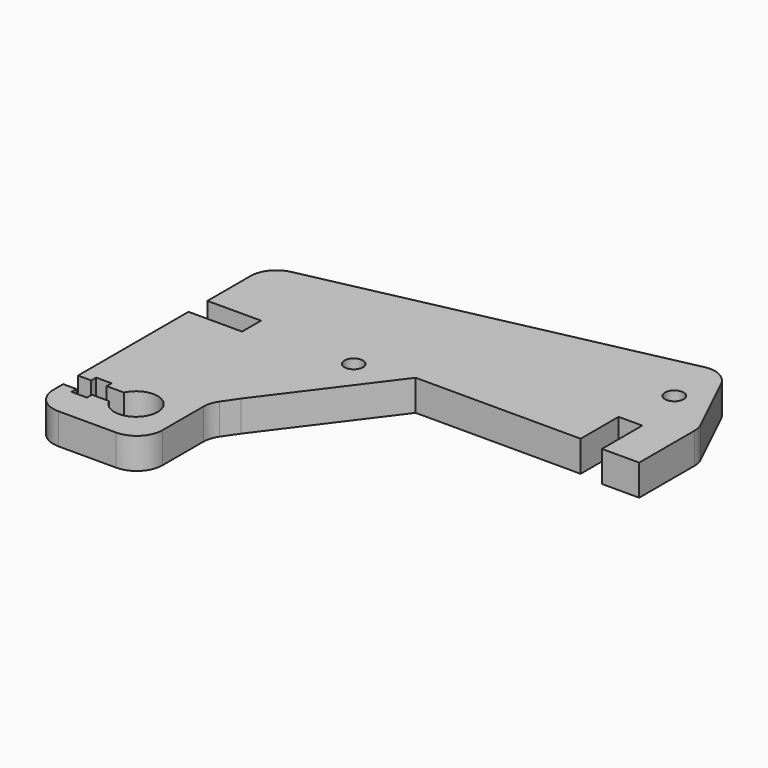
from build123d import *

# Parameters (mm, degrees)
F0_R     = 1.8
F1_DEPTH = 6


# Not quite as in the source:
# - a feature names something its author has since deleted; it is built from what else it names


with BuildPart() as f1:
    # F0 (on Top) → F1 (new body)
    with BuildSketch(Plane.XY):
        with BuildLine():
            ThreePointArc((-26.9197331922, -29.0044), (-22.202470707, -26.7069691338), (-18.925, -30.8044))
            ThreePointArc((-18.925, -30.8044), (-22.202470707, -34.9018308662), (-26.9197331922, -32.6044))
            Line((-26.9197331922, -32.6044), (-30.2622788846, -32.6044))
            Line((-30.2622788846, -32.6044), (-30.2622788846, -33.8044))
            Line((-30.2622788846, -33.8044), (-33.2622788846, -33.8044))
            Line((-33.2622788846, -33.8044), (-33.2622788846, -32.6044))
            Line((-33.2622788846, -32.6044), (-35.8254, -32.6044))
            Line((-35.8254, -32.6044), (-35.8254, -35.0044))
            ThreePointArc((-35.8254, -35.0044), (-34.3609339059, -38.5399339059), (-30.8254, -40.0044))
            Line((-30.8254, -40.0044), (-19.625, -40.0044))
            ThreePointArc((-19.625, -40.0044), (-16.0894660941, -38.5399339059), (-14.625, -35.0044))
            Line((-14.625, -35.0044), (-14.625, -25.0977827265))
            ThreePointArc((-14.625, -25.0977827265), (-14.400006794, -23.6147756066), (-13.7452759529, -22.2652350973))
            Line((-13.7452759529, -22.2652350973), (-11.8023123147, -19.4389644026))
            Line((-11.8023123147, -19.4389644026), (4.5746, 2.4))
            Line((4.5746, 2.4), (36.6099, 2.4))
            Line((36.6099, 2.4), (36.6099, 11.6009423509))
            Line((36.6099, 11.6009423509), (37.1099, 11.6009423509))
            Line((37.1099, 11.6009423509), (38.9099, 11.6009423509))
            Line((38.9099, 11.6009423509), (40.7099, 11.6009423509))
            Line((40.7099, 11.6009423509), (41.2099, 11.6009423509))
            Line((41.2099, 11.6009423509), (41.2099, 1.8140082314))
            Line((41.2099, 1.8140082314), (48.4484305441, 1.8140082314))
            Line((48.4484305441, 1.8140082314), (48.4484305441, 15.1736566274))
            ThreePointArc((48.4484305441, 15.1736566274), (48.3232531582, 16.2854589848), (47.9539887514, 17.341592337))
            Line((47.9539887514, 17.341592337), (41.9726020282, 29.7725357096))
            ThreePointArc((41.9726020282, 29.7725357096), (40.1857248711, 31.8008808947), (37.6042192016, 32.6027179373))
            ThreePointArc((37.6042192016, 32.6027179373), (37.1447174672, 32.5688699786), (36.6902824172, 32.4928679158))
            Line((36.6902824172, 32.4928679158), (-31.8765121651, 17.7491195886))
            ThreePointArc((-31.8765121651, 17.7491195886), (-34.7148447435, 16.0028605187), (-35.8254, 12.8608516729))
            Line((-35.8254, 12.8608516729), (-35.8254, 2.4))
            Line((-35.8254, 2.4), (-25.4254, 2.4))
            Line((-25.4254, 2.4), (-25.4254, 1.9))
            Line((-25.4254, 1.9), (-25.4254, -1.7))
            Line((-25.4254, -1.7), (-25.4254, -2.2))
            Line((-25.4254, -2.2), (-35.8254, -2.2))
            Line((-35.8254, -2.2), (-35.8254, -29.0044))
            Line((-35.8254, -29.0044), (-33.2622788846, -29.0044))
            Line((-33.2622788846, -29.0044), (-33.2622788846, -27.8044))
            Line((-33.2622788846, -27.8044), (-30.2622788846, -27.8044))
            Line((-30.2622788846, -27.8044), (-30.2622788846, -29.0044))
            Line((-30.2622788846, -29.0044), (-26.9197331922, -29.0044))
        make_face()
        with Locations((-5.5901, 0.1)):
            Circle(F0_R, mode=Mode.SUBTRACT)
        with Locations((38.9099, 22.2547)):
            Circle(F0_R, mode=Mode.SUBTRACT)
    extrude(amount=F1_DEPTH)


solid = f1.part
